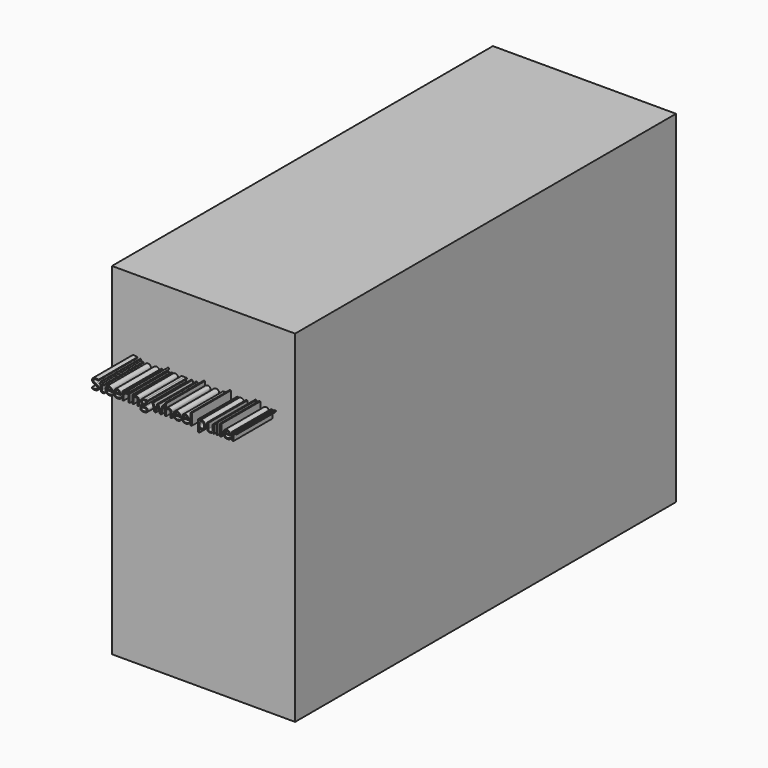
from build123d import *

# Parameters (mm, degrees)
F0_W         = 95.25
F0_H         = 177.8
F1_DEPTH     = 247.65
F2_TEXT_SIZE = 7.7080402725
F3_DEPTH     = 25.4


# Not quite as in the source:
# - Text() gives the source's letters only with a copy of the font that has no kerning and outlines rounded to 1/6400 em; it was checked with that copy


with BuildPart() as f1:
    # F0 (on Front) → F1 (new body)
    with BuildSketch(Plane.XZ):
        Rectangle(F0_W, F0_H)
    extrude(amount=F1_DEPTH)

    # F2 (on face) → F3 (join)
    with BuildSketch(Plane.XZ.offset(247.65)):
        with Locations((-38.1, 46.1587731425)):
            Text('Steering wheel puller', F2_TEXT_SIZE, font='Open Sans', text_align=(TextAlign.LEFT, TextAlign.BOTTOM))
    extrude(amount=F3_DEPTH)


solid = f1.part
